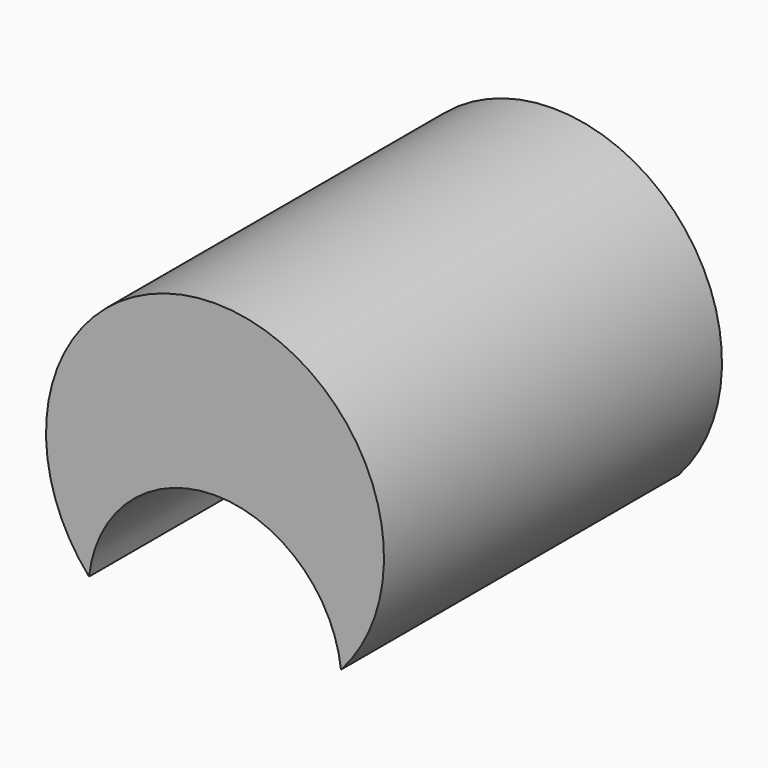
from build123d import *

# Parameters (mm, degrees)
F3_DEPTH = 127


# Not quite as in the source:
# - the program builds the solid bodies; features that only make, move or delete a surface that nothing else refers to are left out


with BuildPart() as f3:
    # F0 (on Front) → F3 (new body)
    with BuildSketch(Plane.XZ):
        with BuildLine():
            ThreePointArc((37.864084419, -48.0037012958), (47.4559558353, -32.2635967896), (50.8, -14.1370346291))
            ThreePointArc((50.8, -14.1370346291), (-18.1265621605, 33.3189212062), (-37.864084419, -48.0037012958))
            ThreePointArc((-37.864084419, -48.0037012958), (0, -14.1370346291), (37.864084419, -48.0037012958))
        make_face()
    extrude(amount=F3_DEPTH)


solid = f3.part
